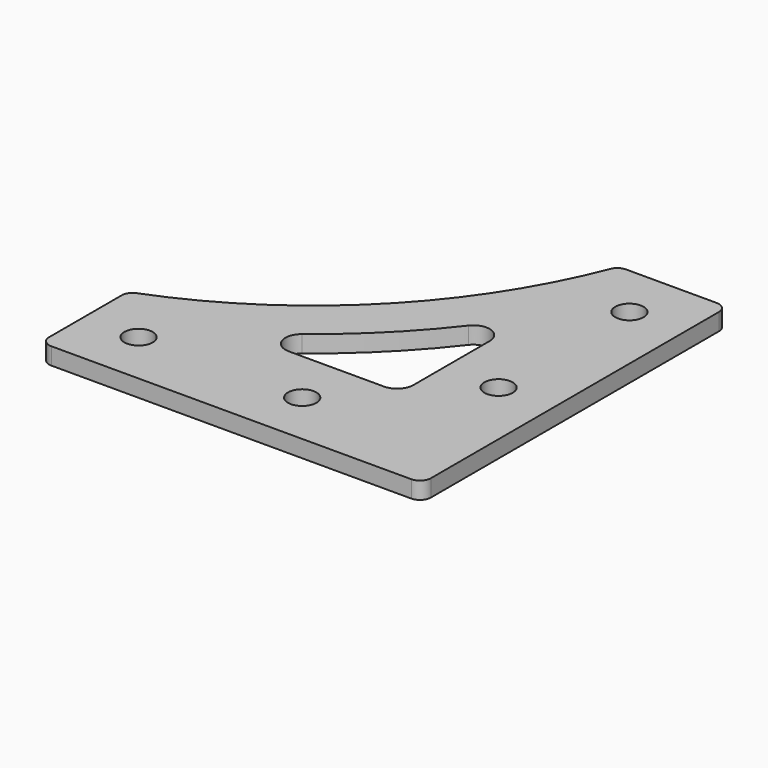
from build123d import *

# Parameters (mm, degrees)
F1_DEPTH = 3.125
F2_W     = 5.9
F2_H     = 50.05
F2_W_2   = 50.05
F2_H_2   = 5.9
F3_DEPTH = 2
F4_R     = 2.6
F5_DEPTH = 25
F6_R     = 2
F8_DEPTH = 25
F9_R     = 3


# Not quite as in the source:
# - a feature names something its author has since deleted; it is built from what else it names


with BuildPart() as f1:
    # F0 (on Top) → F1 (new body)
    with BuildSketch(Plane.XY):
        with BuildLine():
            Line((35, 35), (15, 35))
            ThreePointArc((15, 35), (-4.5539513718, 4.5539513718), (-35, -15))
            Line((-35, -15), (-35, -35))
            Line((-35, -35), (35, -35))
            Line((35, -35), (35, 35))
        make_face()
    extrude(amount=F1_DEPTH)

    # F2 (on face) → F3 (join)
    with BuildSketch(Plane(origin=(0, 0, 0), x_dir=(1, 0, 0), z_dir=(0, 0, -1))):
        with Locations((25, -9.975)):
            Rectangle(F2_W, F2_H)
        with Locations((-9.975, 25)):
            Rectangle(F2_W_2, F2_H_2)
    extrude(amount=F3_DEPTH)

    # F4 (on face) → F5 (cut)
    with BuildSketch(Plane(origin=(0, 0, -2), x_dir=(1, 0, 0), z_dir=(0, 0, -1))):
        with Locations((25, -25)):
            Circle(F4_R)
        with Locations((25, 5)):
            Circle(F4_R)
        with Locations((5, 25)):
            Circle(F4_R)
        with Locations((-25, 25)):
            Circle(F4_R)
    extrude(amount=-F5_DEPTH, mode=Mode.SUBTRACT)

    # F6
    f6_edges = [f1.edges().sort_by_distance(p)[0] for p in [
        (35, 35, 1.5625),
        (15, 35, 1.5625),
        (-35, -15, 1.5625),
        (-35, -35, 1.5625),
        (35, -35, 1.5625),
    ]]
    fillet(f6_edges, radius=F6_R)

    # F7 (on Top) → F8 (cut)
    with BuildSketch(Plane.XY):
        with BuildLine():
            Line((15, -15), (15, 15))
            ThreePointArc((15, 15), (1.6961399442, -1.6961399442), (-15, -15))
            Line((-15, -15), (15, -15))
        make_face()
    extrude(amount=F8_DEPTH, mode=Mode.SUBTRACT)

    # F9
    f9_edges = [f1.edges().sort_by_distance(p)[0] for p in [
        (15, 15, 1.5625),
        (15, -15, 1.5625),
        (-15, -15, 1.5625),
    ]]
    fillet(f9_edges, radius=F9_R)


solid = f1.part
